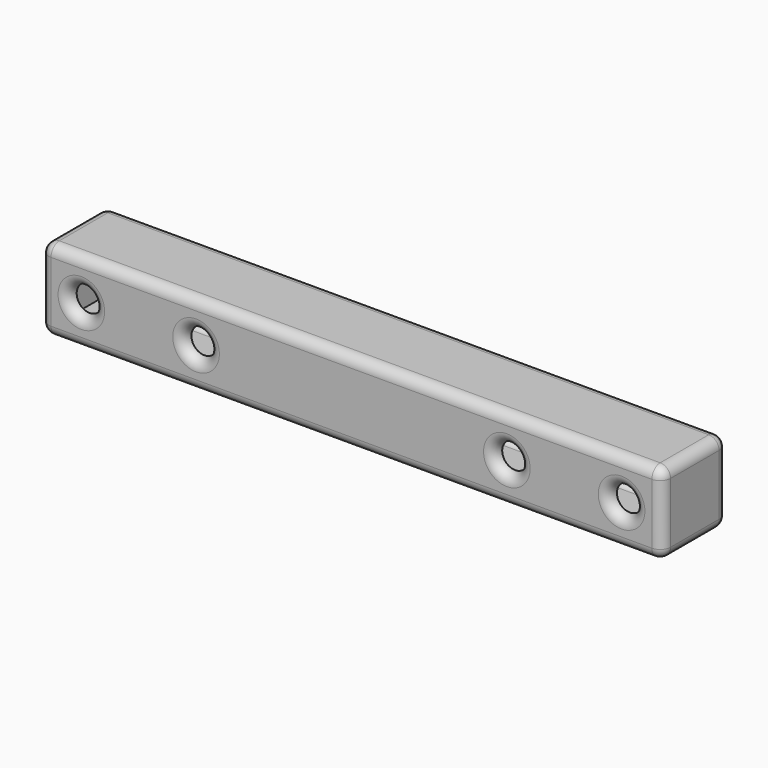
from build123d import *

# Parameters (mm, degrees)
F0_R     = 6.35
F1_DEPTH = 39.878
F2_R     = 5.08
F3_R     = 5.08
F4_T     = 2.54
F5_R     = 5.08


# Not quite as in the source:
# - a shell that OpenCascade refuses in one call is made with other operations: the cavity is built on its own and cut out


with BuildPart() as f1:
    # F0 (on Front) → F1 (new body)
    with BuildSketch(Plane.XZ):
        Polygon((-112.522, -19.939), (152.4, -19.939), (152.4, 19.939), (76.2, 19.939), (0, 19.939), (-76.2, 19.939), (-112.522, 19.939), (-152.4, 19.939), (-152.4, -19.939), align=None)
        with Locations((-132.461, 0)):
            Circle(F0_R, mode=Mode.SUBTRACT)
        with Locations((-76.2, 0)):
            Circle(F0_R, mode=Mode.SUBTRACT)
        with Locations((76.2, 0)):
            Circle(F0_R, mode=Mode.SUBTRACT)
        with Locations((132.461, 0)):
            Circle(F0_R, mode=Mode.SUBTRACT)
    extrude(amount=F1_DEPTH)

    # F2
    f2_edges = [f1.edges().sort_by_distance(p)[0] for p in [
        (-138.811, -39.878, 0),
        (-82.55, -39.878, 0),
        (69.85, -39.878, 0),
    ]]
    fillet(f2_edges, radius=F2_R)

    # F3
    f3_edges = [f1.edges().sort_by_distance(p)[0] for p in [
        (126.111, -39.878, 0),
        (126.111, 0, 0),
        (69.85, 0, 0),
        (-82.55, 0, 0),
        (-138.811, 0, 0),
        (0, 0, -19.939),
        (0, 0, 19.939),
        (0, -39.878, 19.939),
        (0, -39.878, -19.939),
    ]]
    fillet(f3_edges, radius=F3_R)

    # F4: shell of thickness 2.54, made by hand


with BuildPart() as f4_core1:
    # F4_t2: copy of F1
    add(f1.part)

    # the walls: a layer under each face that stays
    f4_faces = [f4_core1.faces().sort_by_distance(p)[0] for p in [
        (0, -39.878, 0),
        (152.4, -19.939, 0),
        (0, -38.3901024484, -18.4511024484),
        (0, -38.3901024484, 18.4511024484),
        (-152.4, -19.939, 0),
        (-140.2988975516, -38.3901024484, 0),
        (-84.0378975516, -38.3901024484, 0),
        (68.3621024484, -38.3901024484, 0),
        (124.6231024484, -38.3901024484, 0),
        (0, -19.939, -19.939),
        (0, -1.4878975516, -18.4511024484),
        (0, 0, 0),
        (0, -1.4878975516, 18.4511024484),
        (0, -19.939, 19.939),
        (124.6231024484, -1.4878975516, 0),
        (68.3621024484, -1.4878975516, 0),
        (-84.0378975516, -1.4878975516, 0),
        (-140.2988975516, -1.4878975516, 0),
    ]]
    thicken(f4_faces, amount=-F4_T, mode=Mode.SUBTRACT)


with BuildPart() as f1_1:
    add(f1.part)

    # what is left inside the walls is the cavity
    f4_cavity = [f4_core1.part.solids().sort_by_distance(p)[0] for p in [
        (0, -24.892, -17.3736),
    ]]
    add(f4_cavity, mode=Mode.SUBTRACT)

    # F5
    f5_edges = [f1_1.edges().sort_by_distance(p)[0] for p in [
        (-152.4, -19.939, 19.939),
        (152.4, -19.939, -19.939),
        (152.4, -1.487898, -18.451102),
        (152.4, -38.390102, -18.451102),
        (152.4, 0, 0),
        (152.4, -39.878, 0),
        (152.4, -1.487898, 18.451102),
        (152.4, -38.390102, 18.451102),
        (152.4, -19.939, 19.939),
    ]]
    fillet(f5_edges, radius=F5_R)


solid = f1_1.part
